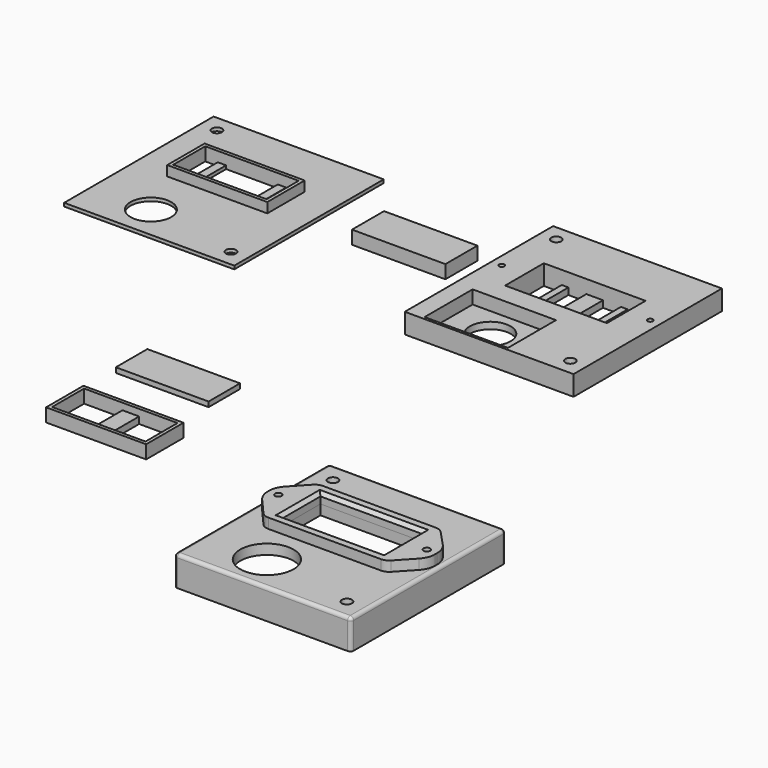
from build123d import *

# Parameters (mm, degrees)
F0_W      = 51
F0_H      = 56
F0_R      = 1.5
F0_R_2    = 6.1
F0_W_2    = 5
F0_H_2    = 14.5
F1_DEPTH  = 1
F0_W_3    = 2.5
F0_H_3    = 12
F3_W      = 28
F3_H      = 1
F4_DEPTH  = 3
F5_W      = 28
F5_H      = 12
F6_DEPTH  = 4
F7_T      = -1
F8_W      = 2
F8_H      = 10
F9_DEPTH  = 3
F2_W      = 30
F2_H      = 14
F11_DEPTH = 4
F2_W_2    = 51
F2_H_2    = 56
F2_R      = 8
F2_R_2    = 1.5
F2_R_3    = 0.8
F2_W_3    = 30.5
F2_H_3    = 14.5
F12_DEPTH = 3
F2_W_4    = 5
F2_H_4    = 2
F2_H_5    = 5
F13_DEPTH = 2
F5_W_2    = 27.8
F5_H_2    = 11.8
F14_DEPTH = 1.5
F2_H_6    = 1
F15_DEPTH = 9
F16_W     = 36.5
F16_H     = 20.5
F16_W_2   = 30.5
F16_H_2   = 14.5
F16_R     = 1
F17_DEPTH = 3
F18_R     = 6
F19_R     = 3
F20_R     = 1
F21_SIZE  = 1
F24_DEPTH = 1
F25_D     = 1.4
F25_DEPTH = 1.001
F27_D     = 1.4
F22_W     = 51
F22_H     = 56
F22_W_2   = 25
F22_H_2   = 18
F22_R     = 1.5
F28_DEPTH = 5
F29_W     = 0.2
F29_H     = 55.6
F30_DEPTH = 25
F31_D     = 1.6
F31_DEPTH = 5.001
F32_D     = 1.6
F33_W     = 2
F33_H     = 14.5
F34_DEPTH = 2


# Not quite as in the source:
# - a feature names something its author has since deleted; it is built from what else it names


with BuildPart() as f1:
    # F0 (on Top) → F1 (new body)
    with BuildSketch(Plane.XY):
        Rectangle(F0_W, F0_H)
        with Locations((20.5, -23)):
            Circle(F0_R, mode=Mode.SUBTRACT)
        with Locations((-7.5, -18)):
            Circle(F0_R_2, mode=Mode.SUBTRACT)
        Polygon((-15.25, -2.75), (-15.25, 11.75), (-2.5, 11.75), (2.5, 11.75), (15.25, 11.75), (15.25, -2.75), (2.5, -2.75), (-2.5, -2.75), align=None, mode=Mode.SUBTRACT)
        with Locations((-20.5, 23)):
            Circle(F0_R, mode=Mode.SUBTRACT)
        with Locations((0, 4.5)):
            Rectangle(F0_W_2, F0_H_2)
    extrude(amount=F1_DEPTH)

    # F24 (add): a face of the model
    f24_faces = [f1.faces().sort_by_distance(p)[0] for p in [
        (0.3722548806, 0.1869472989, 1),
    ]]
    extrude(f24_faces, amount=F24_DEPTH)

    # F25 (through all, one way)
    with BuildSketch(Plane.XY.offset(1)):
        with Locations((-22.25, 4.75), (22.25, 4.75)):
            Circle(F25_D / 2)
    extrude(amount=-F25_DEPTH, mode=Mode.SUBTRACT)

    # F27 (through all)
    with Locations(Plane(origin=(0, 0, 1), x_dir=(1, 0, 0), z_dir=(0, 0, -1))):
        with Locations((-22.25, -4.75), (22.25, -4.75)):
            Hole(F27_D / 2)

    # F22 (on face) → F28 (join)
    with BuildSketch(Plane.XY.offset(1)):
        Rectangle(F22_W, F22_H)
        with Locations((-7.5, -18)):
            Rectangle(F22_W_2, F22_H_2, mode=Mode.SUBTRACT)
        with Locations((20.5, -23)):
            Circle(F22_R, mode=Mode.SUBTRACT)
        with Locations((-20.5, 23)):
            Circle(F22_R, mode=Mode.SUBTRACT)
        Polygon((-15.25, -2.75), (-15.25, 11.75), (-2.5, 11.75), (2.5, 11.75), (15.25, 11.75), (15.25, -2.75), (2.5, -2.75), (-2.5, -2.75), align=None, mode=Mode.SUBTRACT)
    extrude(amount=F28_DEPTH)

    # F29 (on face) → F30 (cut)
    with BuildSketch(Plane(origin=(0, 0, 0), x_dir=(1, 0, 0), z_dir=(0, 0, -1))):
        Polygon((25.5, 28), (-25.5, 28), (-25.5, 27.8), (-25.3, 27.8), (25.3, 27.8), (25.5, 27.8), align=None)
        with Locations((-25.4, 0)):
            Rectangle(F29_W, F29_H)
        with Locations((25.4, 0)):
            Rectangle(F29_W, F29_H)
        Polygon((-25.3, -27.8), (-25.5, -27.8), (-25.5, -28), (25.5, -28), (25.5, -27.8), (25.3, -27.8), align=None)
    extrude(amount=-F30_DEPTH, mode=Mode.SUBTRACT)

    # F31 (through all, one way)
    with BuildSketch(Plane(origin=(0, 0, 1), x_dir=(1, 0, 0), z_dir=(0, 0, -1))):
        with Locations((-22.25, -4.75), (22.25, -4.75)):
            Circle(F31_D / 2)
    extrude(amount=-F31_DEPTH, mode=Mode.SUBTRACT)

    # F32 (through all)
    with Locations(Plane.XY.offset(1)):
        with Locations((22.25, 4.75), (-22.25, 4.75)):
            Hole(F32_D / 2)

    # F33 (on face) → F34 (join)
    with BuildSketch(Plane(origin=(0, 0, 0), x_dir=(1, 0, 0), z_dir=(0, 0, -1))):
        with Locations((-8.875, -4.5)):
            Rectangle(F33_W, F33_H)
        with Locations((8.875, -4.5)):
            Rectangle(F33_W, F33_H)
    extrude(amount=-F34_DEPTH)


with BuildPart() as f1b:
    # F0 (on Top) → F1, piece 2 (new body)
    with BuildSketch(Plane.XY):
        with Locations((-102.5748546124, 1.0383715183)):
            Rectangle(F0_W, F0_H)
        with Locations((-110.0748546124, -16.9616284817)):
            Circle(F0_R_2, mode=Mode.SUBTRACT)
        with Locations((-82.0748546124, -21.9616284817)):
            Circle(F0_R, mode=Mode.SUBTRACT)
        Polygon((-116.5748546124, -0.4616284817), (-116.5748546124, 11.5383715183), (-112.8248546124, 11.5383715183), (-110.3248546124, 11.5383715183), (-94.8248546124, 11.5383715183), (-92.3248546124, 11.5383715183), (-88.5748546124, 11.5383715183), (-88.5748546124, -0.4616284817), (-92.3248546124, -0.4616284817), (-94.8248546124, -0.4616284817), (-110.3248546124, -0.4616284817), (-112.8248546124, -0.4616284817), align=None, mode=Mode.SUBTRACT)
        with Locations((-123.0748546124, 24.0383715183)):
            Circle(F0_R, mode=Mode.SUBTRACT)
        with Locations((-111.5748546124, 5.5383715183)):
            Rectangle(F0_W_3, F0_H_3)
        with Locations((-93.5748546124, 5.5383715183)):
            Rectangle(F0_W_3, F0_H_3)
    extrude(amount=F1_DEPTH)

    # F3 (on face) → F4 (join)
    with BuildSketch(Plane.XY.offset(1)):
        with Locations((-102.5748546124, 12.0383715183)):
            Rectangle(F3_W, F3_H)
        Polygon((-116.5748546124, -0.4616284817), (-116.5748546124, 11.5383715183), (-116.5748546124, 12.5383715183), (-117.5748546124, 12.5383715183), (-117.5748546124, -1.4616284817), (-116.5748546124, -1.4616284817), align=None)
        Polygon((-88.5748546124, 12.5383715183), (-88.5748546124, 11.5383715183), (-88.5748546124, -0.4616284817), (-88.5748546124, -1.4616284817), (-87.5748546124, -1.4616284817), (-87.5748546124, 12.5383715183), align=None)
        with Locations((-102.5748546124, -0.9616284817)):
            Rectangle(F3_W, F3_H)
    extrude(amount=F4_DEPTH)


with BuildPart() as f6:
    # F5 (on Top) → F6 (new body)
    with BuildSketch(Plane.XY):
        with Locations((-49.3556470275, 6)):
            Rectangle(F5_W, F5_H)
    extrude(amount=F6_DEPTH)

    # F7
    f7_openings = [f6.faces().sort_by_distance(p)[0] for p in [
        (-49.355647, 6, 0),
    ]]
    offset(amount=F7_T, openings=f7_openings)

    # F8 (on face) → F9 (join)
    with BuildSketch(Plane(origin=(0, 0, 3), x_dir=(1, 0, 0), z_dir=(0, 0, -1))):
        with Locations((-49.3556470275, -6)):
            Rectangle(F8_W, F8_H)
    extrude(amount=F9_DEPTH)


with BuildPart() as f11:
    # F2 (on Top) → F11 (new body)
    with BuildSketch(Plane.XY):
        with Locations((-48.0005137329, -108.0776734079)):
            Rectangle(F2_W, F2_H)
        Polygon((-62.0005137329, -114.0776734079), (-62.0005137329, -102.0776734079), (-50.5005137329, -102.0776734079), (-45.5005137329, -102.0776734079), (-34.0005137329, -102.0776734079), (-34.0005137329, -107.0776734079), (-34.0005137329, -109.0776734079), (-34.0005137329, -114.0776734079), (-45.5005137329, -114.0776734079), (-50.5005137329, -114.0776734079), align=None, mode=Mode.SUBTRACT)
    extrude(amount=F11_DEPTH)

    # F2 (on Top) → F13 (join)
    with BuildSketch(Plane.XY):
        with Locations((-48.0005137329, -108.0776734079)):
            Rectangle(F2_W_4, F2_H_4)
        with Locations((-48.0005137329, -104.5776734079)):
            Rectangle(F2_W_4, F2_H_5)
        with Locations((-48.0005137329, -111.5776734079)):
            Rectangle(F2_W_4, F2_H_5)
    extrude(amount=F13_DEPTH)


with BuildPart() as f12:
    # F2 (on Top) → F12 (new body)
    with BuildSketch(Plane.XY):
        with Locations((28.2103444552, -118.9687541723)):
            Rectangle(F2_W_2, F2_H_2)
        with Locations((20.7103444552, -136.9687541723)):
            Circle(F2_R, mode=Mode.SUBTRACT)
        with Locations((48.7103444552, -141.9687541723)):
            Circle(F2_R_2, mode=Mode.SUBTRACT)
        with Locations((5.9603444552, -114.2187541723)):
            Circle(F2_R_3, mode=Mode.SUBTRACT)
        with Locations((28.2103444552, -114.4687541723)):
            Rectangle(F2_W_3, F2_H_3, mode=Mode.SUBTRACT)
        with Locations((50.4603444552, -114.2187541723)):
            Circle(F2_R_3, mode=Mode.SUBTRACT)
        with Locations((7.7103444552, -95.9687541723)):
            Circle(F2_R_2, mode=Mode.SUBTRACT)
    extrude(amount=-F12_DEPTH)

    # F2 (on Top) → F15 (join)
    with BuildSketch(Plane.XY):
        Polygon((2.7103444552, -146.9687541723), (2.7103444552, -90.9687541723), (2.7103444552, -89.9687541723), (1.7103444552, -89.9687541723), (1.7103444552, -147.9687541723), (2.7103444552, -147.9687541723), align=None)
        with Locations((28.2103444552, -90.4687541723)):
            Rectangle(F2_W_2, F2_H_6)
        with Locations((28.2103444552, -147.4687541723)):
            Rectangle(F2_W_2, F2_H_6)
        Polygon((53.7103444552, -89.9687541723), (53.7103444552, -90.9687541723), (53.7103444552, -146.9687541723), (53.7103444552, -147.9687541723), (54.7103444552, -147.9687541723), (54.7103444552, -89.9687541723), align=None)
    extrude(amount=-F15_DEPTH)

    # F20
    f20_edges = [f12.edges().sort_by_distance(p)[0] for p in [
        (1.710344, -118.968754, 0),
        (28.210344, -89.968754, 0),
        (28.210344, -147.968754, 0),
        (54.710344, -118.968754, 0),
        (54.710344, -147.968754, -4.5),
        (1.710344, -147.968754, -4.5),
        (1.710344, -89.968754, -4.5),
        (54.710344, -89.968754, -4.5),
    ]]
    fillet(f20_edges, radius=F20_R)


with BuildPart() as f14:
    # F5 (on Top) → F14 (new body)
    with BuildSketch(Plane.XY):
        with Locations((-52.0366017878, -79.3675661445)):
            Rectangle(F5_W_2, F5_H_2)
    extrude(amount=F14_DEPTH)


with BuildPart() as f17:
    # F16 (on face) → F17 (new body)
    with BuildSketch(Plane.XY):
        with Locations((28.2103444552, -114.4687541723)):
            Rectangle(F16_W, F16_H)
        with Locations((28.2103444552, -114.4687541723)):
            Rectangle(F16_W_2, F16_H_2, mode=Mode.SUBTRACT)
        Polygon((9.9603444552, -124.7187541723), (9.9603444552, -104.2187541723), (2.9603444552, -111.7187541723), (2.9603444552, -116.7187541723), align=None)
        with Locations((5.9603444552, -114.2187541723)):
            Circle(F16_R, mode=Mode.SUBTRACT)
        Polygon((53.4603444552, -111.7187541723), (46.4603444552, -104.2187541723), (46.4603444552, -124.7187541723), (53.4603444552, -117.2187541723), align=None)
        with Locations((50.4603444552, -114.2187541723)):
            Circle(F16_R, mode=Mode.SUBTRACT)
    extrude(amount=F17_DEPTH)

    # F18
    f18_edges = [f17.edges().sort_by_distance(p)[0] for p in [
        (2.960344, -111.718754, 1.5),
        (2.960344, -116.718754, 1.5),
        (53.460344, -117.218754, 1.5),
        (53.460344, -111.718754, 1.5),
    ]]
    fillet(f18_edges, radius=F18_R)

    # F19
    f19_edges = [f17.edges().sort_by_distance(p)[0] for p in [
        (9.960344, -104.218754, 1.5),
        (9.960344, -124.718754, 1.5),
        (46.460344, -124.718754, 1.5),
        (46.460344, -104.218754, 1.5),
    ]]
    fillet(f19_edges, radius=F19_R)

    # F21
    f21_edges = [f17.edges().sort_by_distance(p)[0] for p in [
        (12.960344, -114.468754, 3),
        (28.210344, -107.218754, 3),
        (43.460344, -114.468754, 3),
        (28.210344, -121.718754, 3),
    ]]
    chamfer(f21_edges, length=F21_SIZE)


solid = Compound([f1.part, f1b.part, f6.part, f11.part, f12.part, f14.part, f17.part])
